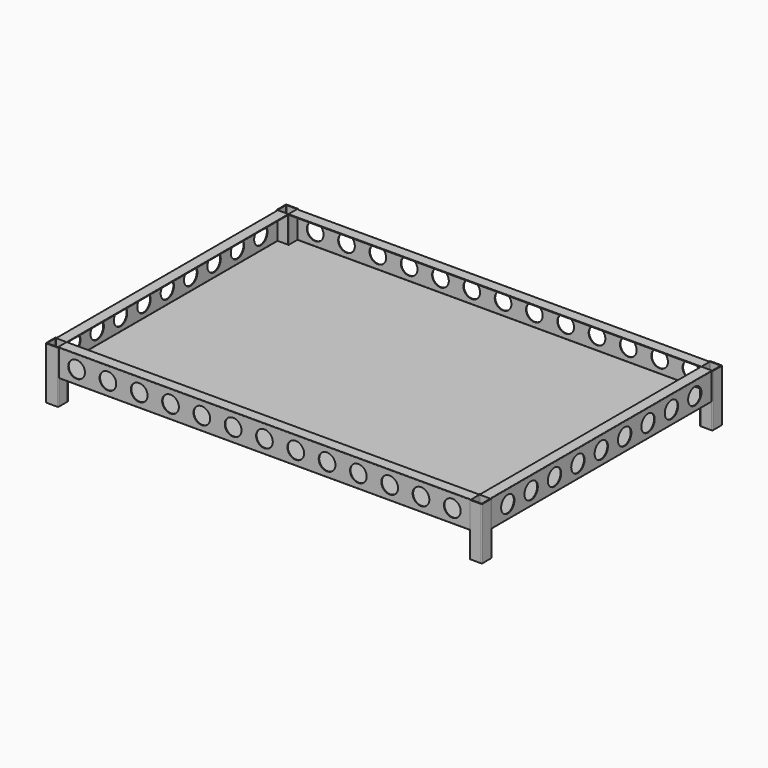
from build123d import *

# Parameters (mm, degrees)
F1_DEPTH  = 125
F3_DEPTH  = 660
F5_DEPTH  = 985
F7_DEPTH  = 985
F8_R      = 20
F9_DEPTH  = 1043.001
F10_R     = 20
F11_DEPTH = 718.001


with BuildPart() as f1:
    # F0 (on Top) → F1 (new body)
    with BuildSketch(Plane.XY):
        with BuildLine():
            Line((-100.4526202679, 26.9756633131), (-74.4526202679, 26.9756633131))
            ThreePointArc((-74.4526202679, 26.9756633131), (-73.0384067055, 27.5614497507), (-72.4526202679, 28.9756633131))
            Line((-72.4526202679, 28.9756633131), (-72.4526202679, 54.9756633131))
            ThreePointArc((-72.4526202679, 54.9756633131), (-73.0384067055, 56.3898768755), (-74.4526202679, 56.9756633131))
            Line((-74.4526202679, 56.9756633131), (-100.4526202679, 56.9756633131))
            ThreePointArc((-100.4526202679, 56.9756633131), (-101.8668338302, 56.3898768755), (-102.4526202679, 54.9756633131))
            Line((-102.4526202679, 54.9756633131), (-102.4526202679, 28.9756633131))
            ThreePointArc((-102.4526202679, 28.9756633131), (-101.8668338302, 27.5614497507), (-100.4526202679, 26.9756633131))
        make_face()
        with BuildLine():
            ThreePointArc((-74.4526202679, 29.9756633131), (-74.7455134867, 29.2685565319), (-75.4526202679, 28.9756633131))
            Line((-75.4526202679, 28.9756633131), (-99.4526202679, 28.9756633131))
            ThreePointArc((-99.4526202679, 28.9756633131), (-100.1597270491, 29.2685565319), (-100.4526202679, 29.9756633131))
            Line((-100.4526202679, 29.9756633131), (-100.4526202679, 53.9756633131))
            ThreePointArc((-100.4526202679, 53.9756633131), (-100.1597270491, 54.6827700943), (-99.4526202679, 54.9756633131))
            Line((-99.4526202679, 54.9756633131), (-75.4526202679, 54.9756633131))
            ThreePointArc((-75.4526202679, 54.9756633131), (-74.7455134867, 54.6827700943), (-74.4526202679, 53.9756633131))
            Line((-74.4526202679, 53.9756633131), (-74.4526202679, 29.9756633131))
        make_face(mode=Mode.SUBTRACT)
    extrude(amount=F1_DEPTH)



with BuildPart() as f1b:
    # F0 (on Top) → F1, piece 2 (new body)
    with BuildSketch(Plane.XY):
        with BuildLine():
            Line((-100.4526202679, -663.0243366869), (-74.4526202679, -663.0243366869))
            ThreePointArc((-74.4526202679, -663.0243366869), (-73.0384067055, -662.4385502493), (-72.4526202679, -661.0243366869))
            Line((-72.4526202679, -661.0243366869), (-72.4526202679, -635.0243366869))
            ThreePointArc((-72.4526202679, -635.0243366869), (-73.0384067055, -633.6101231245), (-74.4526202679, -633.0243366869))
            Line((-74.4526202679, -633.0243366869), (-100.4526202679, -633.0243366869))
            ThreePointArc((-100.4526202679, -633.0243366869), (-101.8668338302, -633.6101231245), (-102.4526202679, -635.0243366869))
            Line((-102.4526202679, -635.0243366869), (-102.4526202679, -661.0243366869))
            ThreePointArc((-102.4526202679, -661.0243366869), (-101.8668338302, -662.4385502493), (-100.4526202679, -663.0243366869))
        make_face()
        with BuildLine():
            Line((-74.4526202679, -636.0243366869), (-74.4526202679, -660.0243366869))
            ThreePointArc((-74.4526202679, -660.0243366869), (-74.7455134867, -660.7314434681), (-75.4526202679, -661.0243366869))
            Line((-75.4526202679, -661.0243366869), (-99.4526202679, -661.0243366869))
            ThreePointArc((-99.4526202679, -661.0243366869), (-100.1597270491, -660.7314434681), (-100.4526202679, -660.0243366869))
            Line((-100.4526202679, -660.0243366869), (-100.4526202679, -636.0243366869))
            ThreePointArc((-100.4526202679, -636.0243366869), (-100.1597270491, -635.3172299057), (-99.4526202679, -635.0243366869))
            Line((-99.4526202679, -635.0243366869), (-75.4526202679, -635.0243366869))
            ThreePointArc((-75.4526202679, -635.0243366869), (-74.7455134867, -635.3172299057), (-74.4526202679, -636.0243366869))
        make_face(mode=Mode.SUBTRACT)
    extrude(amount=F1_DEPTH)


with BuildPart() as f1c:
    # F0 (on Top) → F1, piece 3 (new body)
    with BuildSketch(Plane.XY):
        with BuildLine():
            Line((914.5473797321, -663.0243366869), (940.5473797321, -663.0243366869))
            ThreePointArc((940.5473797321, -663.0243366869), (941.9615932945, -662.4385502493), (942.5473797321, -661.0243366869))
            Line((942.5473797321, -661.0243366869), (942.5473797321, -635.0243366869))
            ThreePointArc((942.5473797321, -635.0243366869), (941.9615932945, -633.6101231245), (940.5473797321, -633.0243366869))
            Line((940.5473797321, -633.0243366869), (914.5473797321, -633.0243366869))
            ThreePointArc((914.5473797321, -633.0243366869), (913.1331661698, -633.6101231245), (912.5473797321, -635.0243366869))
            Line((912.5473797321, -635.0243366869), (912.5473797321, -661.0243366869))
            ThreePointArc((912.5473797321, -661.0243366869), (913.1331661698, -662.4385502493), (914.5473797321, -663.0243366869))
        make_face()
        with BuildLine():
            Line((940.5473797321, -636.0243366869), (940.5473797321, -660.0243366869))
            ThreePointArc((940.5473797321, -660.0243366869), (940.2544865133, -660.7314434681), (939.5473797321, -661.0243366869))
            Line((939.5473797321, -661.0243366869), (915.5473797321, -661.0243366869))
            ThreePointArc((915.5473797321, -661.0243366869), (914.8402729509, -660.7314434681), (914.5473797321, -660.0243366869))
            Line((914.5473797321, -660.0243366869), (914.5473797321, -636.0243366869))
            ThreePointArc((914.5473797321, -636.0243366869), (914.8402729509, -635.3172299057), (915.5473797321, -635.0243366869))
            Line((915.5473797321, -635.0243366869), (939.5473797321, -635.0243366869))
            ThreePointArc((939.5473797321, -635.0243366869), (940.2544865133, -635.3172299057), (940.5473797321, -636.0243366869))
        make_face(mode=Mode.SUBTRACT)
    extrude(amount=F1_DEPTH)


with BuildPart() as f1d:
    # F0 (on Top) → F1, piece 4 (new body)
    with BuildSketch(Plane.XY):
        with BuildLine():
            Line((914.5473797321, 26.9756633131), (940.5473797321, 26.9756633131))
            ThreePointArc((940.5473797321, 26.9756633131), (941.9615932945, 27.5614497507), (942.5473797321, 28.9756633131))
            Line((942.5473797321, 28.9756633131), (942.5473797321, 54.9756633131))
            ThreePointArc((942.5473797321, 54.9756633131), (941.9615932945, 56.3898768755), (940.5473797321, 56.9756633131))
            Line((940.5473797321, 56.9756633131), (914.5473797321, 56.9756633131))
            ThreePointArc((914.5473797321, 56.9756633131), (913.1331661698, 56.3898768755), (912.5473797321, 54.9756633131))
            Line((912.5473797321, 54.9756633131), (912.5473797321, 28.9756633131))
            ThreePointArc((912.5473797321, 28.9756633131), (913.1331661698, 27.5614497507), (914.5473797321, 26.9756633131))
        make_face()
        with BuildLine():
            Line((940.5473797321, 53.9756633131), (940.5473797321, 29.9756633131))
            ThreePointArc((940.5473797321, 29.9756633131), (940.2544865133, 29.2685565319), (939.5473797321, 28.9756633131))
            Line((939.5473797321, 28.9756633131), (915.5473797321, 28.9756633131))
            ThreePointArc((915.5473797321, 28.9756633131), (914.8402729509, 29.2685565319), (914.5473797321, 29.9756633131))
            Line((914.5473797321, 29.9756633131), (914.5473797321, 53.9756633131))
            ThreePointArc((914.5473797321, 53.9756633131), (914.8402729509, 54.6827700943), (915.5473797321, 54.9756633131))
            Line((915.5473797321, 54.9756633131), (939.5473797321, 54.9756633131))
            ThreePointArc((939.5473797321, 54.9756633131), (940.2544865133, 54.6827700943), (940.5473797321, 53.9756633131))
        make_face(mode=Mode.SUBTRACT)
    extrude(amount=F1_DEPTH)


with BuildPart() as f1_1:
    add(f1.part)

    add(f1b.part)  # F3 merges F1b

    add(f1c.part)  # F3 merges F1c

    add(f1d.part)  # F3 merges F1d
    # F2 (on face) → F3 (join, through all)
    with BuildSketch(Plane.XZ.offset(-26.9756633131)):
        with BuildLine():
            Line((-74.4526202679, 123.5), (-74.4526202679, 125))
            Line((-74.4526202679, 125), (-99.4526202679, 125))
            ThreePointArc((-99.4526202679, 125), (-100.1597270491, 124.7071067812), (-100.4526202679, 124))
            Line((-100.4526202679, 124), (-100.4526202679, 61))
            ThreePointArc((-100.4526202679, 61), (-100.1597270491, 60.2928932188), (-99.4526202679, 60))
            Line((-99.4526202679, 60), (939.5473797321, 60))
            ThreePointArc((939.5473797321, 60), (940.2544865133, 60.2928932188), (940.5473797321, 61))
            Line((940.5473797321, 61), (940.5473797321, 124))
            ThreePointArc((940.5473797321, 124), (940.2544865133, 124.7071067812), (939.5473797321, 125))
            Line((939.5473797321, 125), (914.5515561104, 125))
            Line((914.5515561104, 125), (914.5515561104, 123.5))
            Line((914.5515561104, 123.5), (938.5473797321, 123.5))
            ThreePointArc((938.5473797321, 123.5), (938.9009331227, 123.3535533906), (939.0473797321, 123))
            Line((939.0473797321, 123), (939.0473797321, 62))
            ThreePointArc((939.0473797321, 62), (938.9009331227, 61.6464466094), (938.5473797321, 61.5))
            Line((938.5473797321, 61.5), (-98.4526202679, 61.5))
            ThreePointArc((-98.4526202679, 61.5), (-98.8061736585, 61.6464466094), (-98.9526202679, 62))
            Line((-98.9526202679, 62), (-98.9526202679, 123))
            ThreePointArc((-98.9526202679, 123), (-98.8061736585, 123.3535533906), (-98.4526202679, 123.5))
            Line((-98.4526202679, 123.5), (-74.4526202679, 123.5))
        make_face()
    extrude(amount=F3_DEPTH)

    # F4 (on face) → F5 (join, through all)
    with BuildSketch(Plane(origin=(912.5473797321, 0, 0), x_dir=(0, -1, 0), z_dir=(-1, 0, 0))):
        with BuildLine():
            Line((660.0243366869, 125), (635.0243366869, 125))
            Line((635.0243366869, 125), (635.0243366869, 123.5))
            Line((635.0243366869, 123.5), (659.0243366869, 123.5))
            ThreePointArc((659.0243366869, 123.5), (659.3778900775, 123.3535533906), (659.5243366869, 123))
            Line((659.5243366869, 123), (659.5243366869, 62))
            ThreePointArc((659.5243366869, 62), (659.3778900775, 61.6464466094), (659.0243366869, 61.5))
            Line((659.0243366869, 61.5), (633.0243366869, 61.5))
            Line((633.0243366869, 61.5), (633.0243366869, 60))
            Line((633.0243366869, 60), (660.0243366869, 60))
            ThreePointArc((660.0243366869, 60), (660.7314434681, 60.2928932188), (661.0243366869, 61))
            Line((661.0243366869, 61), (661.0243366869, 124))
            ThreePointArc((661.0243366869, 124), (660.7314434681, 124.7071067812), (660.0243366869, 125))
        make_face()
    extrude(amount=F5_DEPTH)

    # F6 (on face) → F7 (join, through all)
    with BuildSketch(Plane(origin=(912.5473797321, 0, 0), x_dir=(0, -1, 0), z_dir=(-1, 0, 0))):
        with BuildLine():
            Line((-28.9756633131, 123.5), (-28.9756633131, 125))
            Line((-28.9756633131, 125), (-53.9756633131, 125))
            ThreePointArc((-53.9756633131, 125), (-54.6827700943, 124.7071067812), (-54.9756633131, 124))
            Line((-54.9756633131, 124), (-54.9756633131, 61))
            ThreePointArc((-54.9756633131, 61), (-54.6827700943, 60.2928932188), (-53.9756633131, 60))
            Line((-53.9756633131, 60), (-26.9756633131, 60))
            Line((-26.9756633131, 60), (-26.9756633131, 61.5))
            Line((-26.9756633131, 61.5), (-52.9756633131, 61.5))
            ThreePointArc((-52.9756633131, 61.5), (-53.3292167037, 61.6464466094), (-53.4756633131, 62))
            Line((-53.4756633131, 62), (-53.4756633131, 123))
            ThreePointArc((-53.4756633131, 123), (-53.3292167037, 123.3535533906), (-52.9756633131, 123.5))
            Line((-52.9756633131, 123.5), (-28.9756633131, 123.5))
        make_face()
    extrude(amount=F7_DEPTH)

    # F8 (on face) → F9 (cut, through all)
    with BuildSketch(Plane(origin=(-100.4526202679, 0, 0), x_dir=(0, -1, 0), z_dir=(-1, 0, 0))):
        with Locations((303.0243366869, 92.5)):
            Circle(F8_R)
        with Locations((373.0243366869, 92.5)):
            Circle(F8_R)
        with Locations((443.0243366869, 92.5)):
            Circle(F8_R)
        with Locations((513.0243366869, 92.5)):
            Circle(F8_R)
        with Locations((583.0243366869, 92.5)):
            Circle(F8_R)
        with Locations((163.0243366869, 92.5)):
            Circle(F8_R)
        with Locations((93.0243366869, 92.5)):
            Circle(F8_R)
        with Locations((23.0243366869, 92.5)):
            Circle(F8_R)
        with Locations((233.0243366869, 92.5)):
            Circle(F8_R)
    extrude(amount=-F9_DEPTH, mode=Mode.SUBTRACT)

    # F10 (on face) → F11 (cut, through all)
    with BuildSketch(Plane(origin=(0, 54.9756633131, 0), x_dir=(-1, 0, 0), z_dir=(0, 1, 0))):
        with Locations((-420.0473797321, 92.5)):
            Circle(F10_R)
        with Locations((-345.0473797321, 92.5)):
            Circle(F10_R)
        with Locations((-270.0473797321, 92.5)):
            Circle(F10_R)
        with Locations((-195.0473797321, 92.5)):
            Circle(F10_R)
        with Locations((-120.0473797321, 92.5)):
            Circle(F10_R)
        with Locations((-45.0473797321, 92.5)):
            Circle(F10_R)
        with Locations((29.9526202679, 92.5)):
            Circle(F10_R)
        with Locations((-645.0473797321, 92.5)):
            Circle(F10_R)
        with Locations((-570.0473797321, 92.5)):
            Circle(F10_R)
        with Locations((-495.0473797321, 92.5)):
            Circle(F10_R)
        with Locations((-720.0473797321, 92.5)):
            Circle(F10_R)
        with Locations((-870.0473797321, 92.5)):
            Circle(F10_R)
        with Locations((-795.0473797321, 92.5)):
            Circle(F10_R)
    extrude(amount=-F11_DEPTH, mode=Mode.SUBTRACT)


solid = f1_1.part
